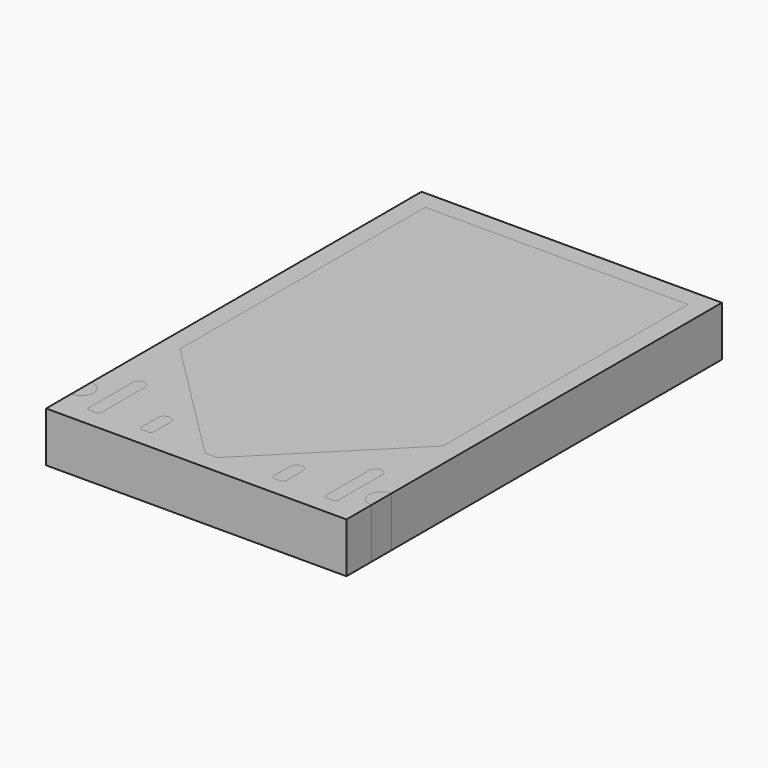
from build123d import *

# Parameters (mm, degrees)
F1_DEPTH = 25.4
F3_DEPTH = 25.4


with BuildPart() as f1:
    # F0 (on Top) → F1 (new body)
    with BuildSketch(Plane.XY):
        with BuildLine():
            Line((76.2, 128.27), (-76.2, 128.27))
            Line((-76.2, 128.27), (-76.2, -81.28))
            ThreePointArc((-76.2, -81.28), (-69.85, -87.63), (-76.2, -93.98))
            Line((-76.2, -93.98), (-76.2, -109.855))
            Line((-76.2, -109.855), (76.2, -109.855))
            Line((76.2, -109.855), (76.2, -93.98))
            ThreePointArc((76.2, -93.98), (69.85, -87.63), (76.2, -81.28))
            Line((76.2, -81.28), (76.2, 128.27))
        make_face()
        with BuildLine():
            Line((-56.9765769958, -71.0984617472), (-56.9765769958, -98.7425))
            ThreePointArc((-56.9765769958, -98.7425), (-57.4415449807, -99.8650320151), (-58.5640769958, -100.33))
            Line((-58.5640769958, -100.33), (-61.7390769958, -100.33))
            ThreePointArc((-61.7390769958, -100.33), (-62.861609011, -99.8650320151), (-63.3265769958, -98.7425))
            Line((-63.3265769958, -98.7425), (-63.3265769958, -71.0984617472))
            ThreePointArc((-63.3265769958, -71.0984617472), (-60.1515769958, -67.9234617472), (-56.9765769958, -71.0984617472))
        make_face(mode=Mode.SUBTRACT)
        with BuildLine():
            Line((-30.3292849183, -88.2243067026), (-30.3292849183, -98.7425))
            ThreePointArc((-30.3292849183, -98.7425), (-30.7942529032, -99.8650320151), (-31.9167849183, -100.33))
            Line((-31.9167849183, -100.33), (-35.0917849183, -100.33))
            ThreePointArc((-35.0917849183, -100.33), (-36.2143169334, -99.8650320151), (-36.6792849183, -98.7425))
            Line((-36.6792849183, -98.7425), (-36.6792849183, -88.2243067026))
            ThreePointArc((-36.6792849183, -88.2243067026), (-33.5042849183, -85.0493067026), (-30.3292849183, -88.2243067026))
        make_face(mode=Mode.SUBTRACT)
        with BuildLine():
            Line((36.6792849183, -88.2243067026), (36.6792849183, -98.7425))
            ThreePointArc((36.6792849183, -98.7425), (36.2143169334, -99.8650320151), (35.0917849183, -100.33))
            Line((35.0917849183, -100.33), (31.9167849183, -100.33))
            ThreePointArc((31.9167849183, -100.33), (30.7942529032, -99.8650320151), (30.3292849183, -98.7425))
            Line((30.3292849183, -98.7425), (30.3292849183, -88.2243067026))
            ThreePointArc((30.3292849183, -88.2243067026), (33.5042849183, -85.0493067026), (36.6792849183, -88.2243067026))
        make_face(mode=Mode.SUBTRACT)
        with BuildLine():
            ThreePointArc((58.5640769958, -100.33), (57.4415449807, -99.8650320151), (56.9765769958, -98.7425))
            Line((56.9765769958, -98.7425), (56.9765769958, -71.0984617472))
            ThreePointArc((56.9765769958, -71.0984617472), (60.1515769958, -67.9234617472), (63.3265769958, -71.0984617472))
            Line((63.3265769958, -71.0984617472), (63.3265769958, -98.7425))
            ThreePointArc((63.3265769958, -98.7425), (62.861609011, -99.8650320151), (61.7390769958, -100.33))
            Line((61.7390769958, -100.33), (58.5640769958, -100.33))
        make_face(mode=Mode.SUBTRACT)
        Polygon((-66.675, 118.745), (66.675, 118.745), (66.675, -36.83), (3.175, -100.33), (0, -100.33), (-3.175, -100.33), (-66.675, -36.83), align=None, mode=Mode.SUBTRACT)
    extrude(amount=F1_DEPTH)


with BuildPart() as f3:
    # F2 (on face) → F3 (new body)
    with BuildSketch(Plane.XY.offset(25.4)):
        Polygon((-66.675, -36.83), (-3.175, -100.33), (3.175, -100.33), (66.675, -36.83), (66.675, 118.745), (-66.675, 118.745), align=None)
    extrude(amount=-F3_DEPTH)


with BuildPart() as f3b:
    # F2 (on face) → F3, piece 2 (new body)
    with BuildSketch(Plane.XY.offset(25.4)):
        with BuildLine():
            Line((-63.3265769958, -71.0984617472), (-63.3265769958, -98.7425))
            ThreePointArc((-63.3265769958, -98.7425), (-62.861609011, -99.8650320151), (-61.7390769958, -100.33))
            Line((-61.7390769958, -100.33), (-58.5640769958, -100.33))
            ThreePointArc((-58.5640769958, -100.33), (-57.4415449807, -99.8650320151), (-56.9765769958, -98.7425))
            Line((-56.9765769958, -98.7425), (-56.9765769958, -71.0984617472))
            ThreePointArc((-56.9765769958, -71.0984617472), (-60.1515769958, -67.9234617472), (-63.3265769958, -71.0984617472))
        make_face()
    extrude(amount=-F3_DEPTH)


with BuildPart() as f3c:
    # F2 (on face) → F3, piece 3 (new body)
    with BuildSketch(Plane.XY.offset(25.4)):
        with BuildLine():
            Line((-76.2, -81.28), (-76.2, -93.98))
            ThreePointArc((-76.2, -93.98), (-69.85, -87.63), (-76.2, -81.28))
        make_face()
    extrude(amount=-F3_DEPTH)


with BuildPart() as f3d:
    # F2 (on face) → F3, piece 4 (new body)
    with BuildSketch(Plane.XY.offset(25.4)):
        with BuildLine():
            Line((-36.6792849183, -88.2243067026), (-36.6792849183, -98.7425))
            ThreePointArc((-36.6792849183, -98.7425), (-36.2143169334, -99.8650320151), (-35.0917849183, -100.33))
            Line((-35.0917849183, -100.33), (-31.9167849183, -100.33))
            ThreePointArc((-31.9167849183, -100.33), (-30.7942529032, -99.8650320151), (-30.3292849183, -98.7425))
            Line((-30.3292849183, -98.7425), (-30.3292849183, -88.2243067026))
            ThreePointArc((-30.3292849183, -88.2243067026), (-33.5042849183, -85.0493067026), (-36.6792849183, -88.2243067026))
        make_face()
    extrude(amount=-F3_DEPTH)


with BuildPart() as f3e:
    # F2 (on face) → F3, piece 5 (new body)
    with BuildSketch(Plane.XY.offset(25.4)):
        with BuildLine():
            Line((30.3292849183, -88.2243067026), (30.3292849183, -98.7425))
            ThreePointArc((30.3292849183, -98.7425), (30.7942529032, -99.8650320151), (31.9167849183, -100.33))
            Line((31.9167849183, -100.33), (35.0917849183, -100.33))
            ThreePointArc((35.0917849183, -100.33), (36.2143169334, -99.8650320151), (36.6792849183, -98.7425))
            Line((36.6792849183, -98.7425), (36.6792849183, -88.2243067026))
            ThreePointArc((36.6792849183, -88.2243067026), (33.5042849183, -85.0493067026), (30.3292849183, -88.2243067026))
        make_face()
    extrude(amount=-F3_DEPTH)


with BuildPart() as f3f:
    # F2 (on face) → F3, piece 6 (new body)
    with BuildSketch(Plane.XY.offset(25.4)):
        with BuildLine():
            ThreePointArc((61.7390769958, -100.33), (62.861609011, -99.8650320151), (63.3265769958, -98.7425))
            Line((63.3265769958, -98.7425), (63.3265769958, -71.0984617472))
            ThreePointArc((63.3265769958, -71.0984617472), (60.1515769958, -67.9234617472), (56.9765769958, -71.0984617472))
            Line((56.9765769958, -71.0984617472), (56.9765769958, -98.7425))
            ThreePointArc((56.9765769958, -98.7425), (57.4415449807, -99.8650320151), (58.5640769958, -100.33))
            Line((58.5640769958, -100.33), (61.7390769958, -100.33))
        make_face()
    extrude(amount=-F3_DEPTH)


with BuildPart() as f3g:
    # F2 (on face) → F3, piece 7 (new body)
    with BuildSketch(Plane.XY.offset(25.4)):
        with BuildLine():
            ThreePointArc((76.2, -81.28), (69.85, -87.63), (76.2, -93.98))
            Line((76.2, -93.98), (76.2, -81.28))
        make_face()
    extrude(amount=-F3_DEPTH)


solid = Compound([f1.part, f3.part, f3b.part, f3c.part, f3d.part, f3e.part, f3f.part, f3g.part])
